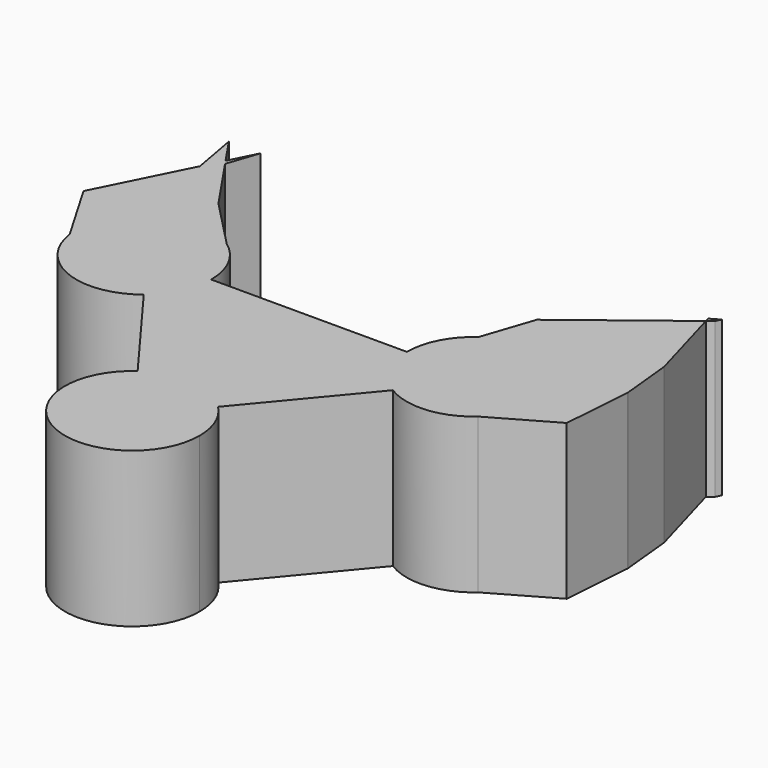
from build123d import *

# Parameters (mm, degrees)
F1_DEPTH = 25.4


with BuildPart() as f1:
    # F0 (on Top) → F1 (new body)
    with BuildSketch(Plane.XY):
        with BuildLine():
            ThreePointArc((-37.8734666786, 33.6277300409), (-34.8188839288, 37.4687345669), (-33.7290209754, 42.2537100409))
            ThreePointArc((-33.7290209754, 42.2537100409), (-33.7290294473, 42.2673925671), (-33.7290548629, 42.2810750723))
            ThreePointArc((-33.7290548629, 42.2810750723), (-34.9562672594, 47.3146936352), (-38.3431132138, 51.2354895473))
            ThreePointArc((-38.3431132138, 51.2354895473), (-50.4880897696, 51.7128598635), (-55.723366114, 40.743802495))
            ThreePointArc((-55.723366114, 40.743802495), (-48.8696733861, 31.9902417407), (-37.8734666786, 33.6277300409))
        make_face()
        with BuildLine():
            ThreePointArc((-33.7290548629, 42.2810750723), (-33.7290294473, 42.2673925671), (-33.7290209754, 42.2537100409))
            ThreePointArc((-33.7290209754, 42.2537100409), (-34.8188839288, 37.4687345669), (-37.8734666786, 33.6277300409))
            Line((-37.8734666786, 33.6277300409), (-25.2242405565, 16.5560153692))
            ThreePointArc((-25.2242405565, 16.5560153692), (-17.8663248029, 18.5222079697), (-10.9841542957, 15.2602198201))
            Line((-10.9841542957, 15.2602198201), (3.627766169, 32.8406458768))
            ThreePointArc((3.627766169, 32.8406458768), (-0.2370073884, 36.8733511802), (-1.6354740563, 42.2810750723))
            Line((-1.6354740563, 42.2810750723), (-33.7290548629, 42.2810750723))
        make_face()
        with BuildLine():
            ThreePointArc((-55.723366114, 40.743802495), (-50.4880897696, 51.7128598635), (-38.3431132138, 51.2354895473))
            Line((-38.3431132138, 51.2354895473), (-46.2101437151, 59.3555606902))
            Line((-46.2101437151, 59.3555606902), (-52.4026783197, 68.4622334303))
            Line((-52.4026783197, 68.4622334303), (-54.0672166674, 63.5277806198))
            Line((-54.0672166674, 63.5277806198), (-54.503296363, 65.9313786952))
            Line((-54.503296363, 65.9313786952), (-60.4510493577, 54.0358843751))
            Line((-60.4510493577, 54.0358843751), (-61.8512481451, 51.2354895473))
            Line((-61.8512481451, 51.2354895473), (-55.723366114, 40.743802495))
        make_face()
        with BuildLine():
            ThreePointArc((2.9785842946, 51.2354895473), (-0.4082616598, 47.3146936352), (-1.6354740563, 42.2810750723))
            ThreePointArc((-1.6354740563, 42.2810750723), (-0.2370073884, 36.8733511802), (3.627766169, 32.8406458768))
            ThreePointArc((3.627766169, 32.8406458768), (10.3472373536, 31.2442359064), (16.7018712654, 33.9494984888))
            ThreePointArc((16.7018712654, 33.9494984888), (19.4785231759, 37.6956896857), (20.4624920562, 42.2537100409))
            ThreePointArc((20.4624920562, 42.2537100409), (14.4623090039, 52.0817234938), (2.9785842946, 51.2354895473))
        make_face()
        with BuildLine():
            ThreePointArc((-10.9841542957, 15.2602198201), (-17.8663248029, 18.5222079697), (-25.2242405565, 16.5560153692))
            ThreePointArc((-25.2242405565, 16.5560153692), (-23.9590672402, -2.2873187943), (-7.8186062971, 7.5186705217))
            ThreePointArc((-7.8186062971, 7.5186705217), (-8.6405670833, 11.7005444937), (-10.9841542957, 15.2602198201))
        make_face()
        with BuildLine():
            Line((5.8138054379, 59.6403814852), (2.9785842946, 51.2354895473))
            ThreePointArc((2.9785842946, 51.2354895473), (14.4623090039, 52.0817234938), (20.4624920562, 42.2537100409))
            ThreePointArc((20.4624920562, 42.2537100409), (19.4785231759, 37.6956896857), (16.7018712654, 33.9494984888))
            Line((16.7018712654, 33.9494984888), (26.7032850534, 39.661302415))
            Line((26.7032850534, 39.661302415), (27.5560012574, 51.1132045745))
            Line((27.5560012574, 51.1132045745), (26.7032850534, 59.6403814852))
            Line((26.7032850534, 59.6403814852), (22.9439260349, 72.8916155568))
            Line((22.9439260349, 72.8916155568), (5.8138054379, 59.6403814852))
        make_face()
        Polygon((-54.0672166674, 63.5277806198), (-52.4026783197, 68.4622334303), (-52.8839736318, 69.1700209806), (-54.503296363, 65.9313786952), align=None)
        Polygon((-52.8839736318, 69.1700209806), (-52.4026783197, 68.4622334303), (-50.6707469221, 73.596470058), align=None)
        Polygon((-54.503296363, 65.9313786952), (-52.8839736318, 69.1700209806), (-55.8939576149, 73.596470058), align=None)
    extrude(amount=F1_DEPTH)


with BuildPart() as f1b:
    # F0 (on Top) → F1, piece 2 (new body)
    with BuildSketch(Plane.XY):
        Polygon((22.7439596686, 73.596470058), (22.9439260349, 72.8916155568), (23.8551047631, 73.596470058), align=None)
        Polygon((22.7439596686, 73.596470058), (23.8551047631, 73.596470058), (24.3033679332, 74.4929955189), align=None)
    extrude(amount=F1_DEPTH)


with BuildPart() as f1c:
    # F0 (on Top) → F1, piece 3 (new body)
    with BuildSketch(Plane.XY):
        Polygon((27.5577381253, 51.1365305556), (27.5560012574, 51.1132045745), (27.5577381253, 51.0958358645), align=None)
    extrude(amount=F1_DEPTH)


solid = Compound([f1.part, f1b.part, f1c.part])
